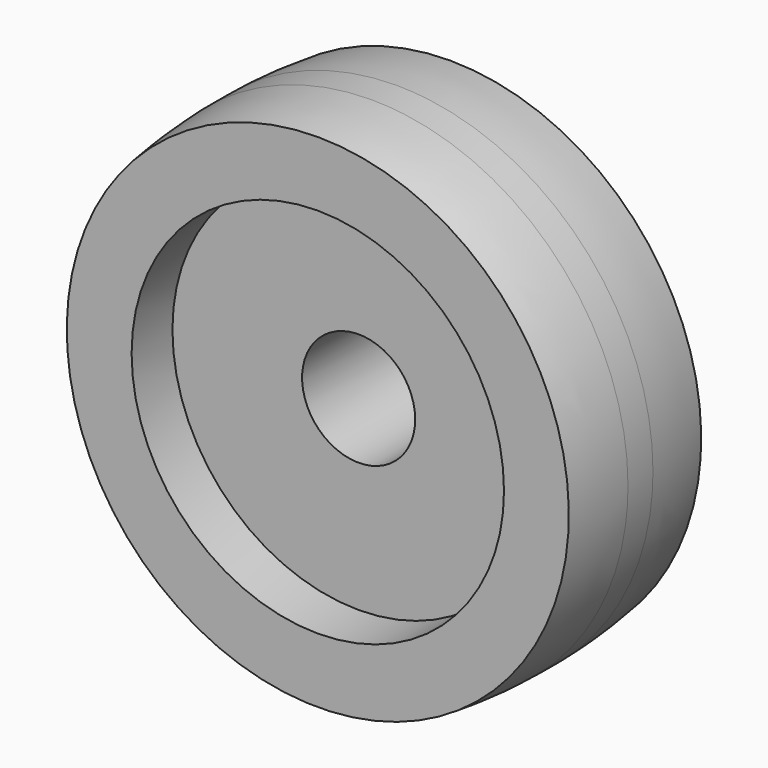
from build123d import *

# Parameters (mm, degrees)
F0_R     = 18.6
F0_R_2   = 4.1
F1_DEPTH = 12
F2_R     = 13.5
F2_R_2   = 4.1
F3_DEPTH = 3.7
F5_DEPTH = 4.2


# Not quite as in the source:
# - ends of sketch curves that miss each other by under 0.0002 mm in the source are joined


with BuildPart() as f1:
    # F0 (on Front) → F1 (new body)
    with BuildSketch(Plane.XZ):
        Circle(F0_R)
        Circle(F0_R_2, mode=Mode.SUBTRACT)
    extrude(amount=F1_DEPTH)

    # F2 (on face) → F3 (cut)
    with BuildSketch(Plane.XZ.offset(12)):
        Circle(F2_R)
        Circle(F2_R_2, mode=Mode.SUBTRACT)
    extrude(amount=-F3_DEPTH, mode=Mode.SUBTRACT)

    # F4 (on face) → F5 (cut)
    with BuildSketch(Plane(origin=(0, 0, 0), x_dir=(-1, 0, 0), z_dir=(0, 1, 0))):
        with BuildLine():
            Line((-7.4463871349, 3.4338489537), (-12.3084865507, 6.2402851562))
            ThreePointArc((-12.3084865507, 6.2402851562), (-13.3297808283, 3.5716863063), (-13.7796064717, 0.7499636563))
            Line((-13.7796064717, 0.7499636563), (-8.1665450744, 0.7399605041))
            ThreePointArc((-8.1665450744, 0.7399605041), (-7.9218161925, 2.1177412996), (-7.4463871349, 3.4338489537))
        make_face()
        with BuildLine():
            Line((-0.75, 8.1656291858), (-0.75, 13.7796044936))
            ThreePointArc((-0.75, 13.7796044936), (-3.5717111631, 13.3297741679), (-6.2402985973, 12.3084797362))
            Line((-6.2402985973, 12.3084797362), (-3.4376390894, 7.4446381706))
            ThreePointArc((-3.4376390894, 7.4446381706), (-2.1246263899, 7.9199723928), (-0.75, 8.1656291858))
        make_face()
        with BuildLine():
            ThreePointArc((6.2402985973, 12.3084797362), (3.5717111631, 13.3297741679), (0.75, 13.7796044936))
            Line((0.75, 13.7796044936), (0.75, 8.1656291858))
            ThreePointArc((0.75, 8.1656291858), (2.1246263899, 7.9199723928), (3.4376390894, 7.4446381706))
            Line((3.4376390894, 7.4446381706), (6.2402985973, 12.3084797362))
        make_face()
        with BuildLine():
            Line((7.5393145037, 11.5584919784), (4.7304979814, 6.6979391493))
            ThreePointArc((4.7304979814, 6.6979391493), (5.7956887156, 5.8008613423), (6.6937164195, 4.7364713126))
            Line((6.6937164195, 4.7364713126), (11.5584775515, 7.5393366214))
            ThreePointArc((11.5584775515, 7.5393366214), (9.7580642441, 9.7580829166), (7.5393145037, 11.5584919784))
        make_face()
        with BuildLine():
            Line((12.3084865507, 6.2402851562), (7.4463871349, 3.4338489537))
            ThreePointArc((7.4463871349, 3.4338489537), (7.9218161925, 2.1177412996), (8.1665450744, 0.7399605041))
            Line((8.1665450744, 0.7399605041), (13.7796064717, 0.7499636563))
            ThreePointArc((13.7796064717, 0.7499636563), (13.3297808283, 3.5716863063), (12.3084865507, 6.2402851562))
        make_face()
        with BuildLine():
            ThreePointArc((-6.6937164195, 4.7364713126), (-5.7956887156, 5.8008613423), (-4.7304979814, 6.6979391493))
            Line((-4.7304979814, 6.6979391493), (-7.5393145037, 11.5584919784))
            ThreePointArc((-7.5393145037, 11.5584919784), (-9.7580642441, 9.7580829166), (-11.5584775515, 7.5393366214))
            Line((-11.5584775515, 7.5393366214), (-6.6937164195, 4.7364713126))
        make_face()
        with BuildLine():
            Line((-8.1665450744, -0.7399605041), (-13.7796064717, -0.7499636563))
            ThreePointArc((-13.7796064717, -0.7499636563), (-13.3297808283, -3.5716863063), (-12.3084865507, -6.2402851562))
            Line((-12.3084865507, -6.2402851562), (-7.4463871349, -3.4338489537))
            ThreePointArc((-7.4463871349, -3.4338489537), (-7.9218161925, -2.1177412996), (-8.1665450744, -0.7399605041))
        make_face()
        with BuildLine():
            ThreePointArc((-4.7304979814, -6.6979391493), (-5.7956887156, -5.8008613423), (-6.6937164195, -4.7364713126))
            Line((-6.6937164195, -4.7364713126), (-11.5584775515, -7.5393366214))
            ThreePointArc((-11.5584775515, -7.5393366214), (-9.7580642441, -9.7580829166), (-7.5393145037, -11.5584919784))
            Line((-7.5393145037, -11.5584919784), (-4.7304979814, -6.6979391493))
        make_face()
        with BuildLine():
            ThreePointArc((-0.75, -8.1656291858), (-2.1246263899, -7.9199723928), (-3.4376390894, -7.4446381706))
            Line((-3.4376390894, -7.4446381706), (-6.2402985973, -12.3084797362))
            ThreePointArc((-6.2402985973, -12.3084797362), (-3.5717111631, -13.3297741679), (-0.75, -13.7796044936))
            Line((-0.75, -13.7796044936), (-0.75, -8.1656291858))
        make_face()
        with BuildLine():
            Line((0.75, -8.1656291858), (0.75, -13.7796044936))
            ThreePointArc((0.75, -13.7796044936), (3.5717111631, -13.3297741679), (6.2402985973, -12.3084797362))
            Line((6.2402985973, -12.3084797362), (3.4376390894, -7.4446381706))
            ThreePointArc((3.4376390894, -7.4446381706), (2.1246263899, -7.9199723928), (0.75, -8.1656291858))
        make_face()
        with BuildLine():
            ThreePointArc((6.6937164195, -4.7364713126), (5.7956887156, -5.8008613423), (4.7304979814, -6.6979391493))
            Line((4.7304979814, -6.6979391493), (7.5393145037, -11.5584919784))
            ThreePointArc((7.5393145037, -11.5584919784), (9.7580642441, -9.7580829166), (11.5584775515, -7.5393366214))
            Line((11.5584775515, -7.5393366214), (6.6937164195, -4.7364713126))
        make_face()
        with BuildLine():
            ThreePointArc((8.1665450744, -0.7399605041), (7.9218161925, -2.1177412996), (7.4463871349, -3.4338489537))
            Line((7.4463871349, -3.4338489537), (12.3084865507, -6.2402851562))
            ThreePointArc((12.3084865507, -6.2402851562), (13.3297761181, -3.5717038849), (13.7796044936, -0.75))
            Line((13.7796044936, -0.75), (8.1665450744, -0.7399605041))
        make_face()
    extrude(amount=-F5_DEPTH, mode=Mode.SUBTRACT)

    # F6 (on Right) → F7 (revolve, cut)
    with BuildSketch(Plane.YZ):
        with BuildLine():
            ThreePointArc((-12.0048904791, 18.2), (-6.0048904791, 18.6146934366), (-0.0048904791, 18.2))
            Line((-0.0048904791, 18.2), (0.3708341392, 18.1622945595))
            Line((0.3708341392, 18.1622945595), (0.3708341392, 18.6))
            Line((0.3708341392, 18.6), (0.3567633394, 19.1855213957))
            Line((0.3567633394, 19.1855213957), (-12.2980514625, 19.1855213957))
            Line((-12.2980514625, 19.1855213957), (-12.27635841, 18.5901094228))
            Line((-12.27635841, 18.5901094228), (-12.27635841, 18.1622945595))
            Line((-12.27635841, 18.1622945595), (-12.0048904791, 18.2))
        make_face()
    revolve(axis=Axis((0, -2.5395685887, 0), (0, 1, 0)), mode=Mode.SUBTRACT)


solid = f1.part
